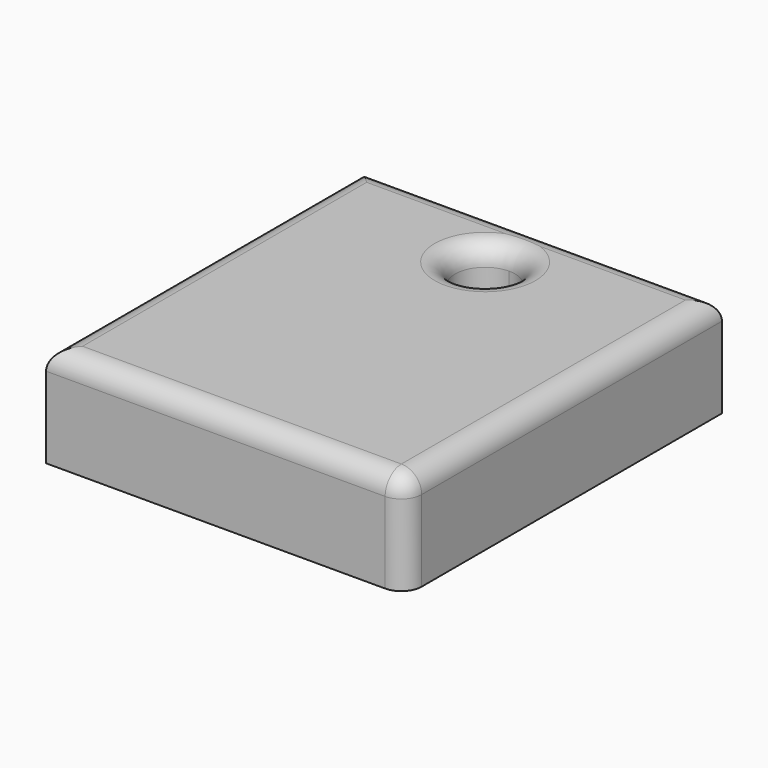
from build123d import *

# Parameters (mm, degrees)
F1_DEPTH     = 25.4
F2_T1_DEPTH  = 97.6486100805
F2_T3_DEPTH  = 106.7304394197
F2_T5_DEPTH  = 33.02
F2_T7_DEPTH  = 115.4286100805
F2_T9_DEPTH  = 124.5104394197
F2_S13_W     = 5.08
F2_S13_H     = 5.08
F2_T14_DEPTH = 5.08


# Not quite as in the source:
# - a fillet or chamfer that OpenCascade refuses, or shapes differently, is made with other operations: its cross-section is extruded or revolved along the edge and cut away or added


with BuildPart() as f1:
    # F0 (on Top) → F1 (new body)
    with BuildSketch(Plane.XY):
        with BuildLine():
            Line((0, 51.6993701458), (-44.1247820854, 51.6993701458))
            Line((-44.1247820854, 51.6993701458), (-44.1247820854, -47.4110692739))
            Line((-44.1247820854, -47.4110692739), (0.8895229548, -47.4110692739))
            Line((0.8895229548, -47.4110692739), (0.8895229548, -45.8316206932))
            Line((0.8895229548, -45.8316206932), (0.223518183, 27.1919083226))
            ThreePointArc((0.223518183, 27.1919083226), (-7.3831209657, 34.6610501168), (0.0860208286, 42.2676892655))
            Line((0.0860208286, 42.2676892655), (0, 51.6993701458))
        make_face()
        with BuildLine():
            Line((45.9038279951, 51.6993701458), (0, 51.6993701458))
            Line((0, 51.6993701458), (0.0860208286, 42.2676892655))
            ThreePointArc((0.0860208286, 42.2676892655), (5.4607226524, 40.0843651019), (7.6929734789, 34.729798794))
            ThreePointArc((7.6929734789, 34.729798794), (5.5093358137, 29.4238456474), (0.223518183, 27.1919083226))
            Line((0.223518183, 27.1919083226), (0.8895229548, -45.8316206932))
            Line((0.8895229548, -45.8316206932), (0.8895229548, -47.4110692739))
            Line((0.8895229548, -47.4110692739), (45.9038279951, -47.4110692739))
            Line((45.9038279951, -47.4110692739), (45.9038279951, 51.6993701458))
        make_face()
    extrude(amount=F1_DEPTH)

    # F2: fillet of radius 5.08 on 8 edges, made by hand

    # F2_s2 → F2_t1 (cut)
    with BuildSketch(Plane.YZ.offset(-56.8247820854)):
        with BuildLine():
            ThreePointArc((-47.4110692739, 20.32), (-45.9231717224, 23.9121024484), (-42.3310692739, 25.4))
            Line((-42.3310692739, 25.4), (-47.4110692739, 25.4))
            Line((-47.4110692739, 25.4), (-47.4110692739, 20.32))
        make_face()
    extrude(amount=F2_T1_DEPTH, mode=Mode.SUBTRACT)

    # F2_s4 → F2_t3 (cut)
    with BuildSketch(Plane.XZ.offset(-64.3993701458)):
        with BuildLine():
            ThreePointArc((45.9038279951, 20.32), (44.4159304435, 23.9121024484), (40.8238279951, 25.4))
            Line((40.8238279951, 25.4), (45.9038279951, 25.4))
            Line((45.9038279951, 25.4), (45.9038279951, 20.32))
        make_face()
    extrude(amount=F2_T3_DEPTH, mode=Mode.SUBTRACT)

    # F2_s6 → F2_t5 (cut)
    with BuildSketch(Plane.XY.offset(-12.7)):
        with BuildLine():
            ThreePointArc((40.8238279951, -47.4110692739), (44.4159304435, -45.9231717224), (45.9038279951, -42.3310692739))
            Line((45.9038279951, -42.3310692739), (45.9038279951, -47.4110692739))
            Line((45.9038279951, -47.4110692739), (40.8238279951, -47.4110692739))
        make_face()
    extrude(amount=F2_T5_DEPTH, mode=Mode.SUBTRACT)

    # F2_s8 → F2_t7 (cut)
    with BuildSketch(Plane.YZ.offset(-56.8247820854)):
        with BuildLine():
            ThreePointArc((51.6993701458, 20.32), (50.2114725942, 23.9121024484), (46.6193701458, 25.4))
            Line((46.6193701458, 25.4), (51.6993701458, 25.4))
            Line((51.6993701458, 25.4), (51.6993701458, 20.32))
        make_face()
    extrude(amount=F2_T7_DEPTH, mode=Mode.SUBTRACT)

    # F2_s10 → F2_t9 (cut)
    with BuildSketch(Plane.XZ.offset(-64.3993701458)):
        with BuildLine():
            ThreePointArc((-44.1247820854, 20.32), (-42.6368845338, 23.9121024484), (-39.0447820854, 25.4))
            Line((-39.0447820854, 25.4), (-44.1247820854, 25.4))
            Line((-44.1247820854, 25.4), (-44.1247820854, 20.32))
        make_face()
    extrude(amount=F2_T9_DEPTH, mode=Mode.SUBTRACT)


with BuildPart() as f2_tool12:
    # F2_s13 → F2_t14 (new body)
    with BuildSketch(Plane.XZ.offset(42.3310692739)):
        with Locations((43.3638279951, 22.86)):
            Rectangle(F2_S13_W, F2_S13_H)
    extrude(amount=F2_T14_DEPTH)

    # F2_s15 → F2_t16 (revolve, cut)
    with BuildSketch(Plane(origin=(40.8238279951, -42.3310692739, 20.32), x_dir=(-0.7071067812, 0, -0.7071067812), z_dir=(-0.7071067812, 0, 0.7071067812))):
        with BuildLine():
            ThreePointArc((0, -5.08), (5.08, 0), (0, 5.08))
            Line((0, 5.08), (0, -5.08))
        make_face()
    revolve(axis=Axis((40.8238279951, -42.3310692739, 20.32), (0, -1, 0)), mode=Mode.SUBTRACT)


with BuildPart() as f1_1:
    add(f1.part)

    # F2_t11: cut F2_tool12
    add(f2_tool12.part, mode=Mode.SUBTRACT)

    # F2_s17 → F2_t18 (revolve, cut)
    with BuildSketch(Plane(origin=(0.4714804091, 0.0043000962, 0), x_dir=(0, 0, 1), z_dir=(-0.9999584116, -0.0091200341, 0))):
        with BuildLine():
            ThreePointArc((20.32, 42.265146908), (23.9121024484, 43.7530444596), (25.4, 47.345146908))
            Line((25.4, 47.345146908), (25.4, 42.265146908))
            Line((25.4, 42.265146908), (20.32, 42.265146908))
        make_face()
    revolve(axis=Axis((0.1547695058, 34.729798794, 25.4), (0, 0, -1)), mode=Mode.SUBTRACT)

    # F2_s19 → F2_t20 (revolve, cut)
    with BuildSketch(Plane(origin=(0.4714804091, 0.0043000962, 0), x_dir=(0, 0, 1), z_dir=(-0.9999584116, -0.0091200341, 0))):
        with BuildLine():
            ThreePointArc((5.08, 42.265146908), (1.4878975516, 43.7530444596), (0, 47.345146908))
            Line((0, 47.345146908), (0, 42.265146908))
            Line((0, 42.265146908), (5.08, 42.265146908))
        make_face()
    revolve(axis=Axis((0.1547695058, 34.729798794, 0), (0, 0, -1)), mode=Mode.SUBTRACT)


solid = f1_1.part
